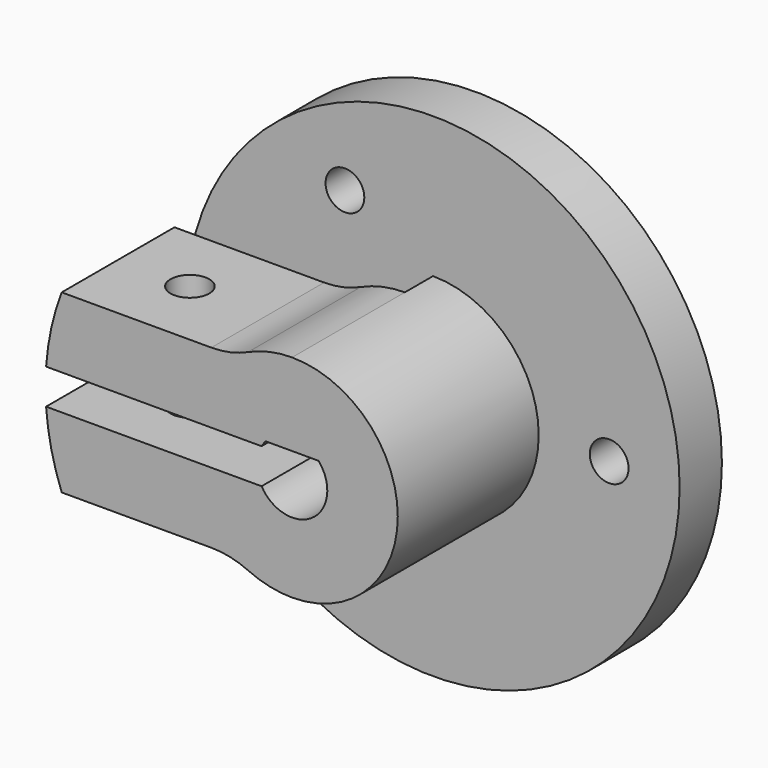
from build123d import *

# Parameters (mm, degrees)
F0_R      = 14
F0_R_2    = 1.1
F1_DEPTH  = 3
F3_DEPTH  = 10
F5_DEPTH  = 13.001
F6_W      = 14
F6_H      = 2
F7_DEPTH  = 6
F8_W      = 14
F8_H      = 2
F9_DEPTH  = 8
F10_R     = 3
F11_DEPTH = 10
F12_R     = 5
F13_R     = 5
F14_R     = 1.1
F15_DEPTH = 19.001


# Not quite as in the source:
# - a feature names something its author has since deleted; it is built from what else it names


with BuildPart() as f1:
    # F0 (on Front) → F1 (new body)
    with BuildSketch(Plane.XZ):
        Circle(F0_R)
        with Locations((-5, -8.6602540378)):
            Circle(F0_R_2, mode=Mode.SUBTRACT)
        with Locations((-5, 8.6602540378)):
            Circle(F0_R_2, mode=Mode.SUBTRACT)
        with Locations((10, 0)):
            Circle(F0_R_2, mode=Mode.SUBTRACT)
    extrude(amount=F1_DEPTH)

    # F2 (on face) → F3 (join)
    with BuildSketch(Plane.XZ.offset(3)):
        with BuildLine():
            ThreePointArc((-3.3166247904, -5), (-1.7320508076, -5.7445626465), (0, -6))
            ThreePointArc((0, -6), (6, 0), (0, 6))
            ThreePointArc((0, 6), (-1.7320508076, 5.7445626465), (-3.3166247904, 5))
            Line((-3.3166247904, 5), (-13.0766968306, 5))
            ThreePointArc((-13.0766968306, 5), (-14, 0), (-13.0766968306, -5))
            Line((-13.0766968306, -5), (-3.3166247904, -5))
        make_face()
    extrude(amount=F3_DEPTH)

    # F4 (on face) → F5 (cut, through all)
    with BuildSketch(Plane(origin=(0, 0, 0), x_dir=(-1, 0, 0), z_dir=(0, 1, 0))):
        with BuildLine():
            Line((1.5, 1.3228756555), (-1.5, 1.3228756555))
            ThreePointArc((-1.5, 1.3228756555), (0, -2), (1.5, 1.3228756555))
        make_face()
    extrude(amount=-F5_DEPTH, mode=Mode.SUBTRACT)

    # F6 (on face) → F7 (cut, symmetric)
    with BuildSketch(Plane.XY.offset(5)):
        with Locations((-7, -4)):
            Rectangle(F6_W, F6_H)
    extrude(amount=F7_DEPTH, both=True, mode=Mode.SUBTRACT)

    # F8 (on face) → F9 (cut)
    with BuildSketch(Plane.XZ.offset(13)):
        with Locations((-7, 0)):
            Rectangle(F8_W, F8_H)
    extrude(amount=-F9_DEPTH, mode=Mode.SUBTRACT)

    # F10 (on face) → F11 (cut)
    with BuildSketch(Plane.XZ.offset(3)):
        with Locations((-5, 8.6602540378)):
            Circle(F10_R)
    extrude(amount=F11_DEPTH, mode=Mode.SUBTRACT)

    # F12
    f12_edges = [f1.edges().sort_by_distance(p)[0] for p in [
        (-3.316625, -9, 5),
    ]]
    fillet(f12_edges, radius=F12_R)

    # F13
    f13_edges = [f1.edges().sort_by_distance(p)[0] for p in [
        (-3.316625, -8, -5),
    ]]
    fillet(f13_edges, radius=F13_R)

    # F14 (on face) → F15 (cut, through all)
    with BuildSketch(Plane.XY.offset(5)):
        with Locations((-9, -9)):
            Circle(F14_R)
    extrude(amount=-F15_DEPTH, mode=Mode.SUBTRACT)


solid = f1.part
